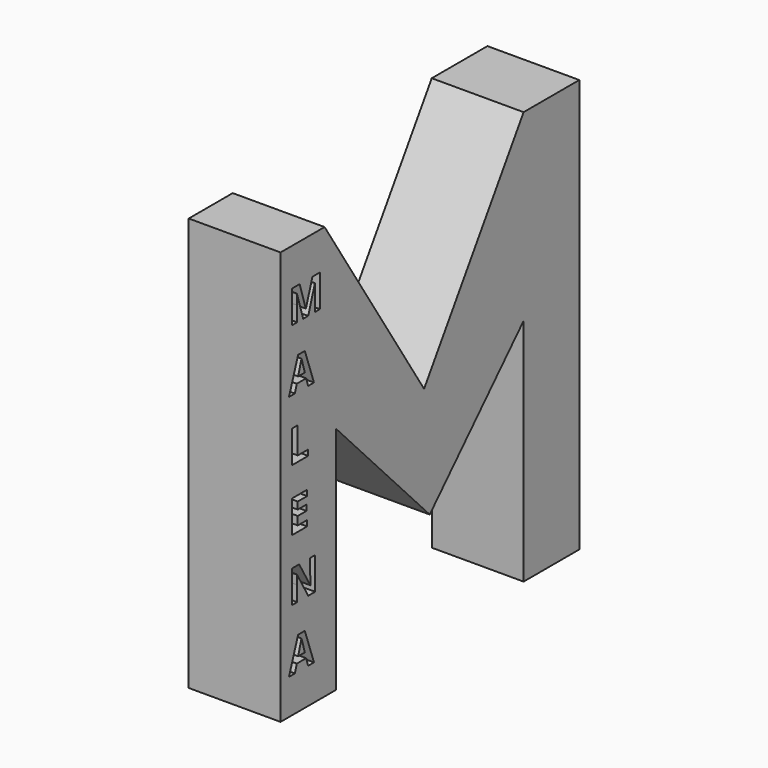
from build123d import *

# Parameters (mm, degrees)
F1_DEPTH     = 25.4
F2_TEXT_SIZE = 12.5260845166
F3_DEPTH     = 6.35


# Not quite as in the source:
# - Text() gives the source's letters only with a copy of the font that has no kerning and outlines rounded to 1/6400 em; it was checked with that copy


with BuildPart() as f1:
    # F0 (on Right) → F1 (new body)
    with BuildSketch(Plane.YZ):
        Polygon((-43.6548526493, 50.8), (-58.8772018308, 50.8), (-58.8772018308, -63.5), (-39.6240018308, -63.5), (-39.6240018308, 0), (-7.3040377054, -33.9879753796), (25.1440381943, 0), (25.1440381943, -63.5), (44.3972381943, -63.5), (44.3972381943, 50.8), (25.1440381943, 50.8), (-9.2554072275, -2.5753515649), align=None)
    extrude(amount=F1_DEPTH)

    # F2 (on face) → F3 (cut)
    with BuildSketch(Plane.YZ.offset(25.4)):
        with Locations((-55.9634511219, 31.4625006215)):
            Text('M', F2_TEXT_SIZE, font='Open Sans', font_style=FontStyle.BOLD, text_align=(TextAlign.LEFT, TextAlign.BOTTOM))
        with Locations((-55.9634511219, 14.4270256789)):
            Text('A', F2_TEXT_SIZE, font='Open Sans', font_style=FontStyle.BOLD, text_align=(TextAlign.LEFT, TextAlign.BOTTOM))
        with Locations((-55.9634511219, -2.6084492637)):
            Text('L', F2_TEXT_SIZE, font='Open Sans', font_style=FontStyle.BOLD, text_align=(TextAlign.LEFT, TextAlign.BOTTOM))
        with Locations((-55.9634511219, -19.6439242063)):
            Text('E', F2_TEXT_SIZE, font='Open Sans', font_style=FontStyle.BOLD, text_align=(TextAlign.LEFT, TextAlign.BOTTOM))
        with Locations((-55.9634511219, -36.6793991489)):
            Text('N', F2_TEXT_SIZE, font='Open Sans', font_style=FontStyle.BOLD, text_align=(TextAlign.LEFT, TextAlign.BOTTOM))
        with Locations((-55.9634511219, -53.7148740915)):
            Text('A', F2_TEXT_SIZE, font='Open Sans', font_style=FontStyle.BOLD, text_align=(TextAlign.LEFT, TextAlign.BOTTOM))
    extrude(amount=-F3_DEPTH, mode=Mode.SUBTRACT)


solid = f1.part
